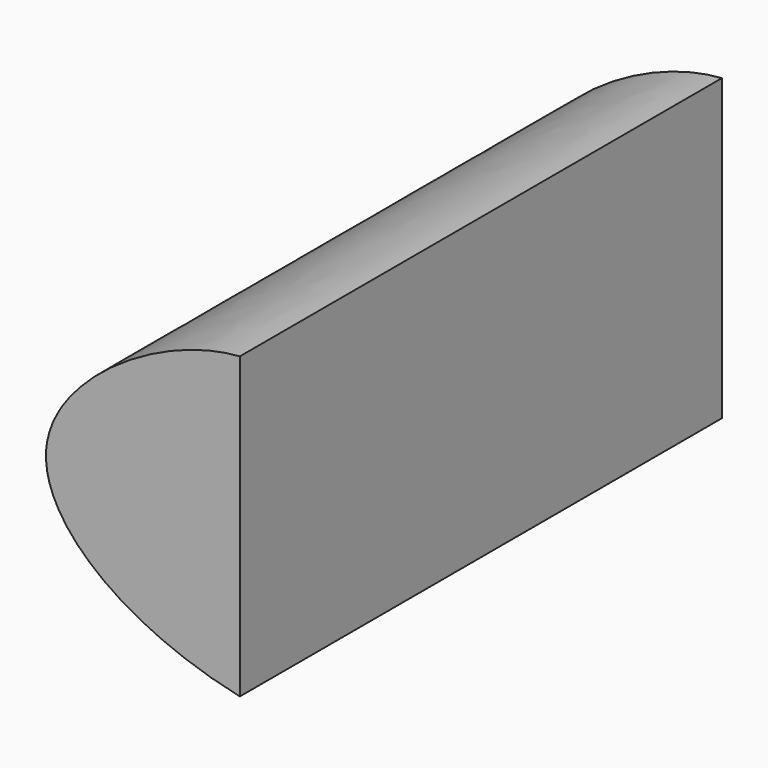
from build123d import *

# Parameters (mm, degrees)
F1_DEPTH = 22.225


# Not quite as in the source:
# - the program builds the solid bodies; features that only make, move or delete a surface that nothing else refers to are left out


with BuildPart() as f1:
    # F0 (on Front) → F1 (new body)
    with BuildSketch(Plane.XZ):
        with BuildLine():
            add(Edge.make_bspline(
                [(0, 0), (-4.3269509836, 0.9381572552), (-7.5359614295, 3.4257399199), (-7.112, 5.9397063551)],
                knots=[0, 0, 0, 0, 0.5071071106, 0.5071071106, 0.5071071106, 0.5071071106], degree=3))
            Line((0, 0), (0, 5.9397063551))
            Line((0, 5.9397063551), (-7.112, 5.9397063551))
        make_face()
        with BuildLine():
            Line((-7.112, 5.9397063551), (0, 5.9397063551))
            Line((0, 5.9397063551), (0, 11.0436904221))
            add(Edge.make_bspline(
                [(-7.112, 5.9397063551), (-6.6999222167, 8.3832062675), (-2.8556827273, 10.8516316045), (0, 11.0436904221)],
                knots=[0.5071071106, 0.5071071106, 0.5071071106, 0.5071071106, 1, 1, 1, 1], degree=3))
        make_face()
    extrude(amount=F1_DEPTH)


solid = f1.part
